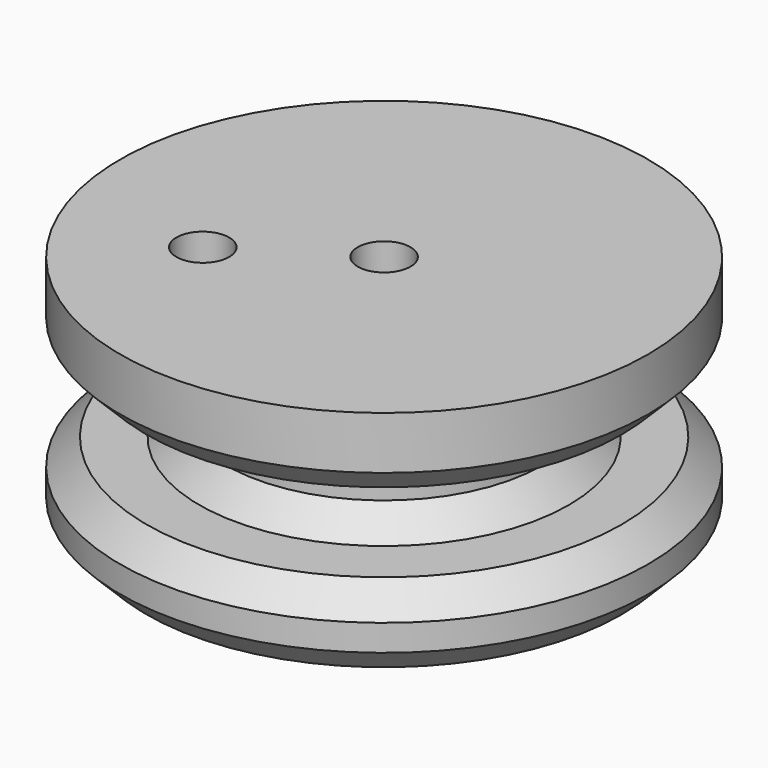
from build123d import *

# Parameters (mm, degrees)
F0_R            = 10
F1_DEPTH        = 3
F2_R            = 6
F3_DEPTH        = 3
F4_R            = 10
F4_R_2          = 6
F5_DEPTH        = 3
F6_SIZE         = 1
F8_D            = 2
F8_DEPTH        = 27
F8_CBORE_D      = 6
F8_CBORE_DEPTH  = 1.2
F8_TIP          = 0.600860619
F10_D           = 2
F10_DEPTH       = 9
F10_CBORE_D     = 3
F10_CBORE_DEPTH = 1.2
F10_TIP         = 0.600860619


with BuildPart() as f1:
    # F0 (on Top) → F1 (new body)
    with BuildSketch(Plane.XY):
        Circle(F0_R)
    extrude(amount=F1_DEPTH)

    # F2 (on face) → F3 (join)
    with BuildSketch(Plane.XY):
        Circle(F2_R)
    extrude(amount=-F3_DEPTH)

    # F4 (on face) → F5 (join)
    with BuildSketch(Plane(origin=(0, 0, -3), x_dir=(1, 0, 0), z_dir=(0, 0, -1))):
        Circle(F4_R)
        Circle(F4_R_2, mode=Mode.SUBTRACT)
        Circle(F4_R_2)
    extrude(amount=F5_DEPTH)

    # F6
    f6_edges = [f1.edges().sort_by_distance(p)[0] for p in [
        (-6, 0, 0),
        (-10, 0, -3),
        (-10, 0, 0),
        (-6, 0, -3),
        (-10, 0, -6),
    ]]
    chamfer(f6_edges, length=F6_SIZE)

    # F8
    with Locations(Plane(origin=(0, 0, -6), x_dir=(1, 0, 0), z_dir=(0, 0, -1))):
        with Locations((0, 0)):
            CounterBoreHole(F8_D / 2, F8_CBORE_D / 2, F8_CBORE_DEPTH, depth=F8_DEPTH)
            with Locations((0, 0, -(F8_DEPTH + F8_TIP / 2))):  # 118° drill point
                Cone(0, F8_D / 2, F8_TIP, mode=Mode.SUBTRACT)

    # F10
    with Locations(Plane(origin=(0, 0, -6), x_dir=(1, 0, 0), z_dir=(0, 0, -1))):
        with Locations((-4.575991758, 2.8671064562)):
            CounterBoreHole(F10_D / 2, F10_CBORE_D / 2, F10_CBORE_DEPTH, depth=F10_DEPTH)
            with Locations((0, 0, -(F10_DEPTH + F10_TIP / 2))):  # 118° drill point
                Cone(0, F10_D / 2, F10_TIP, mode=Mode.SUBTRACT)


solid = f1.part
